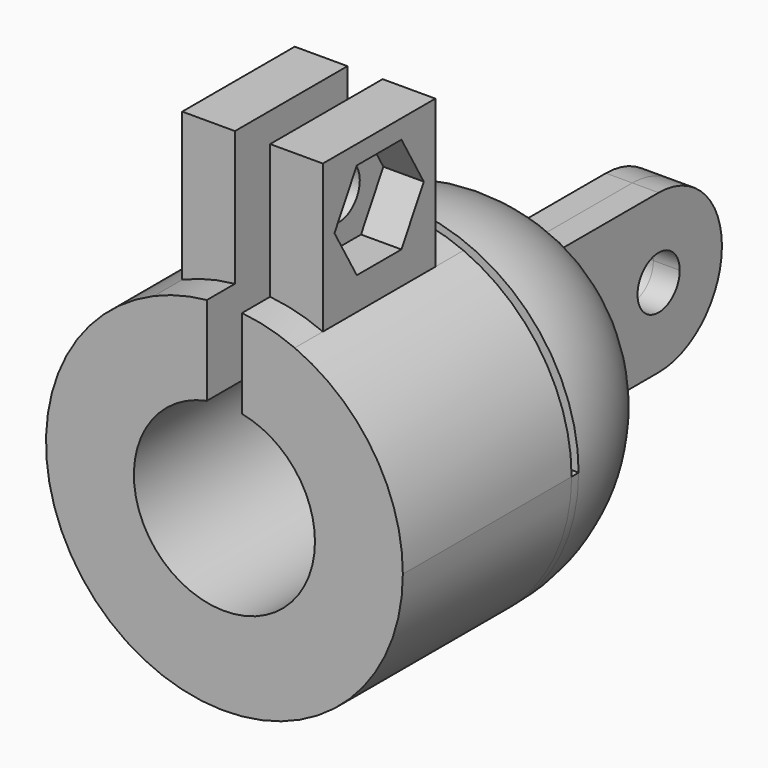
from build123d import *
from build123d import SkipClean  # not in build123d's __all__

# Parameters (mm, degrees)
F1_DEPTH  = 12
F0_W      = 3
F0_H      = 2.5
F2_DEPTH  = 10
F3_DEPTH  = 2
F5_R      = 1.5
F6_DEPTH  = 25
F7_DEPTH  = 2.3
F9_DEPTH  = 0.5
F11_ANGLE = 180
F12_DEPTH = 1.5


with BuildPart() as f1:
    # F0 (on Front) → F1 (new body)
    with BuildSketch(Plane.XZ):
        with BuildLine():
            Line((-4, 9.3285851017), (-1, 9.3285851017))
            Line((-1, 9.3285851017), (-1, 10.1006187929))
            ThreePointArc((-1, 10.1006187929), (-2.529626258, 9.8297248687), (-4, 9.3285851017))
        make_face()
        with BuildLine():
            Line((1, 10.1006187929), (1, 9.3285851017))
            Line((1, 9.3285851017), (4, 9.3285851017))
            ThreePointArc((4, 9.3285851017), (2.529626258, 9.8297248687), (1, 10.1006187929))
        make_face()
        with BuildLine():
            ThreePointArc((1, 5.0519798099), (3.9794786091, 3.2689830223), (5.15, 0))
            ThreePointArc((5.15, 0), (-3.2689830223, -3.9794786091), (-1, 5.0519798099))
            Line((-1, 5.0519798099), (-1, 9.3285851017))
            Line((-1, 9.3285851017), (-4, 9.3285851017))
            ThreePointArc((-4, 9.3285851017), (-5.5867029633, -8.474151875), (10.15, 0))
            ThreePointArc((10.15, 0), (8.474151875, 5.5867029633), (4, 9.3285851017))
            Line((4, 9.3285851017), (1, 9.3285851017))
            Line((1, 9.3285851017), (1, 5.0519798099))
        make_face()
    extrude(amount=F1_DEPTH)

    # F0 (on Front) → F2 (join)
    with BuildSketch(Plane.XZ):
        with BuildLine():
            ThreePointArc((-4, 9.3285851017), (-2.529626258, 9.8297248687), (-1, 10.1006187929))
            Line((-1, 10.1006187929), (-1, 15.2480201901))
            Line((-1, 15.2480201901), (-4, 15.2480201901))
            Line((-4, 15.2480201901), (-4, 9.3285851017))
        make_face()
        with BuildLine():
            Line((1, 15.2480201901), (1, 10.1006187929))
            ThreePointArc((1, 10.1006187929), (2.529626258, 9.8297248687), (4, 9.3285851017))
            Line((4, 9.3285851017), (4, 15.2480201901))
            Line((4, 15.2480201901), (1, 15.2480201901))
        make_face()
        with Locations((-2.5, 16.4980201901)):
            Rectangle(F0_W, F0_H)
        with Locations((2.5, 16.4980201901)):
            Rectangle(F0_W, F0_H)
    extrude(amount=F2_DEPTH)

    # F0 (on Front) → F3 (cut)
    with BuildSketch(Plane.XZ):
        with BuildLine():
            ThreePointArc((-4, 9.3285851017), (-2.529626258, 9.8297248687), (-1, 10.1006187929))
            Line((-1, 10.1006187929), (-1, 15.2480201901))
            Line((-1, 15.2480201901), (-4, 15.2480201901))
            Line((-4, 15.2480201901), (-4, 9.3285851017))
        make_face()
        with BuildLine():
            Line((1, 15.2480201901), (1, 10.1006187929))
            ThreePointArc((1, 10.1006187929), (2.529626258, 9.8297248687), (4, 9.3285851017))
            Line((4, 9.3285851017), (4, 15.2480201901))
            Line((4, 15.2480201901), (1, 15.2480201901))
        make_face()
        with Locations((-2.5, 16.4980201901)):
            Rectangle(F0_W, F0_H)
        with Locations((2.5, 16.4980201901)):
            Rectangle(F0_W, F0_H)
    with SkipClean():  # cleaning this boolean's faces spoils the solid; the shape is the same uncleaned
        extrude(amount=F3_DEPTH, mode=Mode.SUBTRACT)

    # F5 (on face) → F6 (cut)
    with BuildSketch(Plane.YZ.offset(4)):
        with Locations((-6, 13.9243194915)):
            Circle(F5_R)
    extrude(amount=-F6_DEPTH, mode=Mode.SUBTRACT)

    # F5 (on face) → F7 (cut)
    with BuildSketch(Plane.YZ.offset(4)):
        Polygon((-4.4122867597, 16.6743194915), (-7.5877132403, 16.6743194915), (-9.1754264805, 13.9243194915), (-7.5877132403, 11.1743194915), (-4.4122867597, 11.1743194915), (-2.8245735195, 13.9243194915), align=None)
        with Locations((-6, 13.9243194915)):
            Circle(F5_R, mode=Mode.SUBTRACT)
    extrude(amount=-F7_DEPTH, mode=Mode.SUBTRACT)

    # F8 (on face) → F9 (join)
    with BuildSketch(Plane.XZ):
        with BuildLine():
            Line((10.15, 0), (5.15, 0))
            ThreePointArc((5.15, 0), (0, -5.15), (-5.15, 0))
            Line((-5.15, 0), (-10.15, 0))
            ThreePointArc((-10.15, 0), (0, -10.15), (10.15, 0))
        make_face()
        with BuildLine():
            ThreePointArc((-5.15, 0), (0, -5.15), (5.15, 0))
            Line((5.15, 0), (-5.15, 0))
        make_face()
    extrude(amount=-F9_DEPTH)

    # F9_face (on face) → F11 (revolve)
    with BuildSketch(Plane(origin=(0, 0.5, -4.307793793), x_dir=(1, 0, 0), z_dir=(0, 1, 0))):
        with BuildLine():
            Line((-10.15, -4.307793793), (10.15, -4.307793793))
            ThreePointArc((10.15, -4.307793793), (0, 5.842206207), (-10.15, -4.307793793))
        make_face()
    revolve(axis=Axis((0, 0.5, 0), (1, 0, 0)), revolution_arc=F11_ANGLE)

    # F10 (on Right) → F12 (join, symmetric)
    with BuildSketch(Plane.YZ):
        with BuildLine():
            ThreePointArc((17, 4.5), (13.8180194847, 3.1819805153), (12.5, 0))
            Line((12.5, 0), (15.5, 0))
            ThreePointArc((15.5, 0), (15.9393398282, 1.0606601718), (17, 1.5))
            Line((17, 1.5), (17, 4.5))
        make_face()
        with BuildLine():
            ThreePointArc((9.0979393271, 4.5), (9.8834858266, 2.3106726109), (10.15, 0))
            Line((10.15, 0), (12.5, 0))
            ThreePointArc((12.5, 0), (13.8180194847, 3.1819805153), (17, 4.5))
            Line((17, 4.5), (9.0979393271, 4.5))
        make_face()
        with BuildLine():
            Line((12.5, 0), (10.15, 0))
            ThreePointArc((10.15, 0), (9.8834858266, -2.3106726109), (9.0979393271, -4.5))
            Line((9.0979393271, -4.5), (17, -4.5))
            ThreePointArc((17, -4.5), (13.8180194847, -3.1819805153), (12.5, 0))
        make_face()
        with BuildLine():
            Line((15.5, 0), (12.5, 0))
            ThreePointArc((12.5, 0), (13.8180194847, -3.1819805153), (17, -4.5))
            ThreePointArc((17, -4.5), (20.1819805153, -3.1819805153), (21.5, 0))
            ThreePointArc((21.5, 0), (20.1819805153, 3.1819805153), (17, 4.5))
            Line((17, 4.5), (17, 1.5))
            ThreePointArc((17, 1.5), (18.0606601718, 1.0606601718), (18.5, 0))
            ThreePointArc((18.5, 0), (17, -1.5), (15.5, 0))
        make_face()
    extrude(amount=F12_DEPTH, both=True)


solid = f1.part
